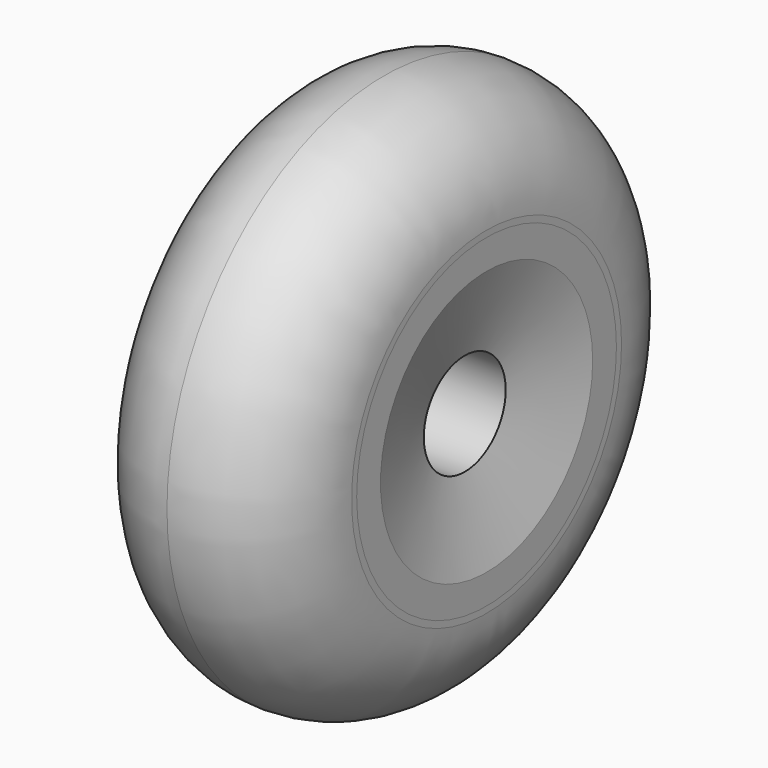
from build123d import *

# Parameters (mm, degrees)
F0_R     = 31.75
F0_R_2   = 18.9992
F1_DEPTH = 24.003
F2_R     = 12.00149
F0_R_3   = 16.002
F3_DEPTH = 24.003
F0_R_4   = 5.9944
F4_DEPTH = 24.003
F5_SIZE2 = 2.5522160579
F5_SIZE  = 9.525
F6_SIZE2 = 2.5522160579
F6_SIZE  = 9.525


# Not quite as in the source:
# - a fillet or chamfer is up to 0.001 mm smaller than in the source, because OpenCascade refuses the exact size


with BuildPart() as f1:
    # F0 (on Right) → F1 (new body)
    with BuildSketch(Plane.YZ):
        Circle(F0_R)
        Circle(F0_R_2, mode=Mode.SUBTRACT)
    extrude(amount=F1_DEPTH)

    # F2 (radius 12.0015 in the source; OpenCascade refuses exactly that, so slightly less here)
    f2_edges = [f1.edges().sort_by_distance(p)[0] for p in [
        (24.003, -31.75, 0),
        (0, -31.75, 0),
    ]]
    fillet(f2_edges, radius=F2_R)


with BuildPart() as f3:
    # F0 (on Right) → F3 (new body)
    with BuildSketch(Plane.YZ):
        Circle(F0_R_2)
        Circle(F0_R_3, mode=Mode.SUBTRACT)
    extrude(amount=F3_DEPTH)

    # F0 (on Right) → F4 (join)
    with BuildSketch(Plane.YZ):
        Circle(F0_R_3)
        Circle(F0_R_4, mode=Mode.SUBTRACT)
    extrude(amount=F4_DEPTH)

    # F5
    f5_edges = [f3.edges().sort_by_distance(p)[0] for p in [
        (24.003, -5.9944, 0),
    ]]
    f5_side = f3.faces().sort_by_distance((24.003, -18.461821, 0))[0]
    chamfer(f5_edges, length=F5_SIZE, length2=F5_SIZE2, reference=f5_side)

    # F6
    f6_edges = [f3.edges().sort_by_distance(p)[0] for p in [
        (0, -5.9944, 0),
    ]]
    f6_side = f3.faces().sort_by_distance((0, -18.461821, 0))[0]
    chamfer(f6_edges, length=F6_SIZE, length2=F6_SIZE2, reference=f6_side)


solid = Compound([f1.part, f3.part])
